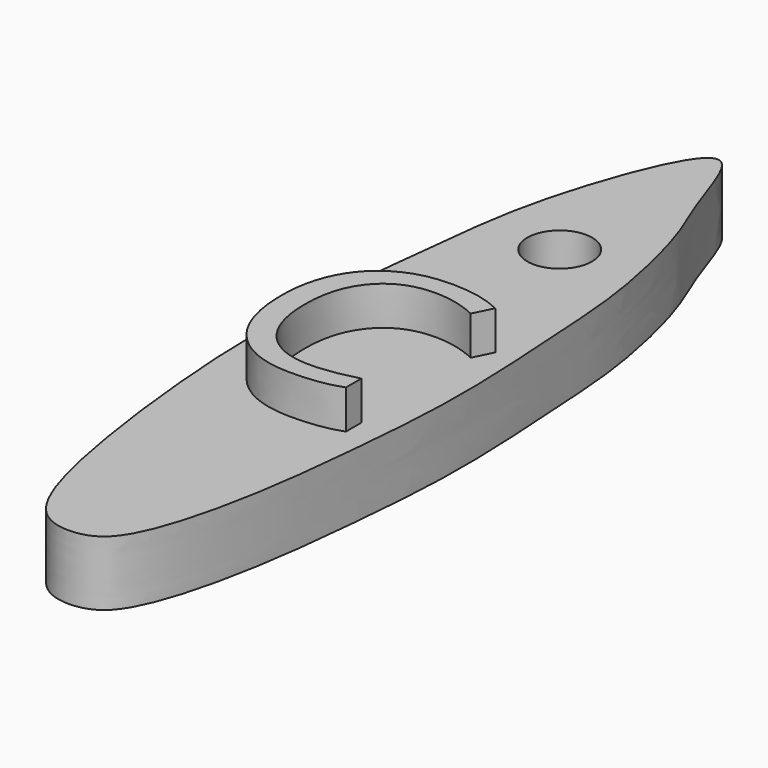
from build123d import *

# Parameters (mm, degrees)
F0_R         = 2.5
F1_DEPTH     = 5
F2_TEXT_SIZE = 20.5973603904
F3_DEPTH     = 3


# Not quite as in the source:
# - Text() gives the source's letters only with a copy of the font that has no kerning and outlines rounded to 1/6400 em; it was checked with that copy


with BuildPart() as f1:
    # F0 (on Top) → F1 (new body)
    with BuildSketch(Plane.XY):
        with BuildLine():
            add(Edge.make_bspline(
                [(-34.6535320873, 65.7954274924), (-33.6588224492, 65.7993400267), (-32.1773452393, 60.563786952), (-30.172806353, 56.596290948), (-28.3613117333, 48.6480291778), (-27.9948988766, 42.329225391), (-27.2961395245, 32.0355434388), (-28.034751624, 23.0424851042), (-29.0480943568, 13.2280696805), (-31.3979990493, 4.7983610845), (-34.206080161, 3.2807910031), (-38.387165041, 3.8503805752), (-40.7208324619, 13.2131759226), (-41.9147460855, 23.5777739205), (-42.3985995884, 33.0678723228), (-40.8354270877, 47.1439256841), (-39.8887354324, 55.5440385457), (-36.04524184, 65.7899534204), (-34.6535320873, 65.7954274924)],
                knots=[0, 0, 0, 0, 0.0501231452, 0.1013987379, 0.1627803286, 0.2199198643, 0.2903240803, 0.3577298156, 0.4288439558, 0.4926785953, 0.5290376695, 0.5687021707, 0.6346747497, 0.7076954332, 0.7769057943, 0.8585366267, 0.9298721281, 1, 1, 1, 1], degree=3))
        make_face()
        with Locations((-34.7039388803, 50.6468183709)):
            Circle(F0_R, mode=Mode.SUBTRACT)
    extrude(amount=F1_DEPTH)

    # F2 (on face) → F3 (join)
    with BuildSketch(Plane.XY.offset(5)):
        with Locations((-41.727515874, 23.6628056638)):
            Text('C', F2_TEXT_SIZE, font='Open Sans', text_align=(TextAlign.LEFT, TextAlign.BOTTOM))
    extrude(amount=F3_DEPTH)


solid = f1.part
